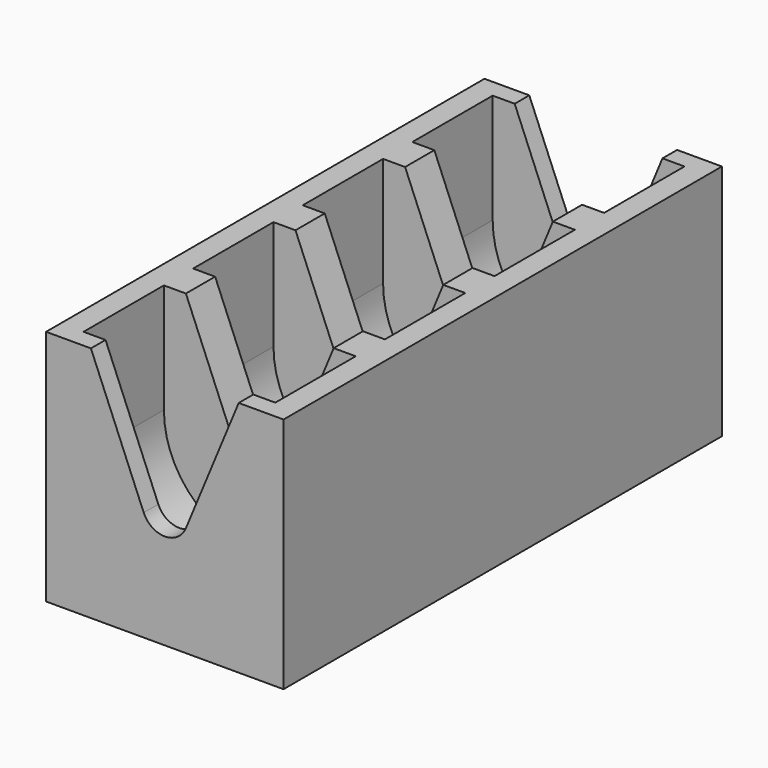
from build123d import *

# Parameters (mm, degrees)
F1_DEPTH = 260
F2_W     = 210
F2_H     = 110
F3_DEPTH = 225
F4_R     = 104.99999
F6_DEPTH = 600.001


# Not quite as in the source:
# - a fillet or chamfer is up to 0.001 mm smaller than in the source, because OpenCascade refuses the exact size


with BuildPart() as f1:
    # F0 (on Top) → F1 (new body)
    with BuildSketch(Plane.XY):
        Polygon((-130, 0), (0, 0), (130, 0), (130, 600), (-130, 600), align=None)
    extrude(amount=F1_DEPTH)

    # F2 (on face) → F3 (cut)
    with BuildSketch(Plane.XY.offset(260)):
        with Locations((0, 525)):
            Rectangle(F2_W, F2_H)
        with Locations((0, 225)):
            Rectangle(F2_W, F2_H)
        with Locations((0, 375)):
            Rectangle(F2_W, F2_H)
        with Locations((0, 75)):
            Rectangle(F2_W, F2_H)
    extrude(amount=-F3_DEPTH, mode=Mode.SUBTRACT)

    # F4 (radius 105 in the source; OpenCascade refuses exactly that, so slightly less here)
    f4_edges = [f1.edges().sort_by_distance(p)[0] for p in [
        (-105, 75, 35),
        (105, 75, 35),
        (-105, 225, 35),
        (-105, 375, 35),
        (-105, 525, 35),
        (105, 225, 35),
        (105, 375, 35),
        (105, 525, 35),
    ]]
    fillet(f4_edges, radius=F4_R)

    # F5 (on face) → F6 (cut, through all)
    with BuildSketch(Plane.XZ):
        with BuildLine():
            ThreePointArc((23.0969883128, 120.4329141909), (24.5196320101, 125.1227419496), (25, 130))
            ThreePointArc((25, 130), (-4.8772580504, 154.5196320101), (-23.0969883128, 120.4329141909))
            ThreePointArc((-23.0969883128, 120.4329141909), (0, 105), (23.0969883128, 120.4329141909))
        make_face()
        with BuildLine():
            ThreePointArc((-23.0969883128, 120.4329141909), (-4.8772580504, 154.5196320101), (25, 130))
            ThreePointArc((25, 130), (24.5196320101, 125.1227419496), (23.0969883128, 120.4329141909))
            Line((23.0969883128, 120.4329141909), (80.9075681158, 260))
            Line((80.9075681158, 260), (0, 260))
            Line((0, 260), (-80.9075681158, 260))
            Line((-80.9075681158, 260), (-23.0969883128, 120.4329141909))
        make_face()
    extrude(amount=-F6_DEPTH, mode=Mode.SUBTRACT)


solid = f1.part
